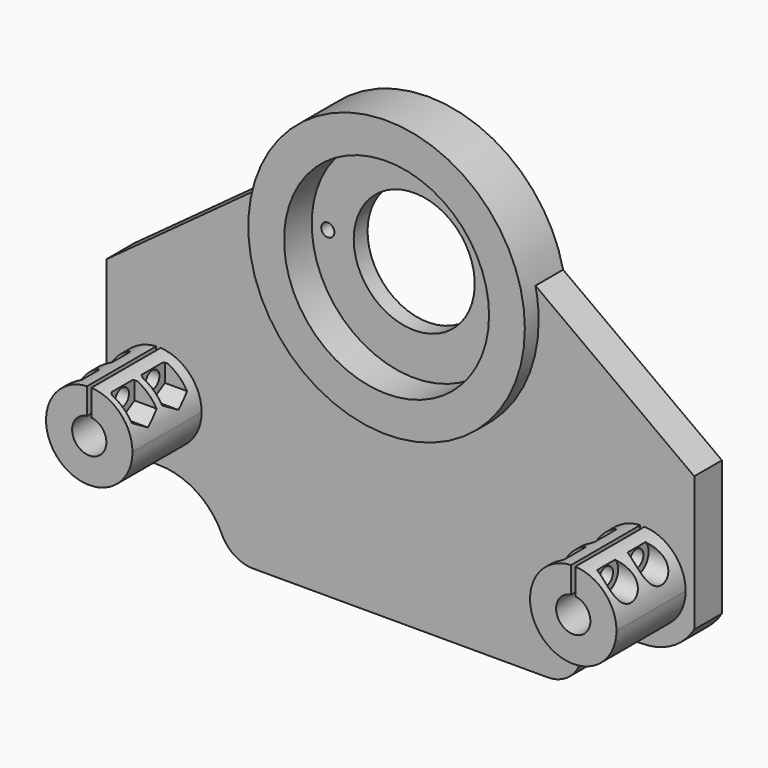
from build123d import *

# Parameters (mm, degrees)
F0_R           = 4.7625
F0_R_2         = 6.2865
F0_R_3         = 37.6555
F1_DEPTH       = 12.7
F2_R           = 63.5
F3_DEPTH       = 25.4
F4_R           = 12.7
F5_R           = 15.875
F5_R_2         = 6.2865
F6_DEPTH       = 31.75
F8_DEPTH       = 31.75
F9_R           = 3.175
F10_DEPTH      = 224.536
F12_DEPTH      = 83.185
F12_DEPTH_BACK = 83.185
F13_R          = 5.55625
F14_DEPTH      = 13.335
F15_R          = 5.55625
F16_DEPTH      = 13.335
F17_W          = 51.1538733715
F17_H          = 19.05
F17_R          = 3.175
F18_DEPTH      = 4.7498
F19_R          = 12.7
F20_R          = 50.8
F20_R_2        = 37.6555
F21_DEPTH      = 12.7
F22_R          = 37.6555
F22_R_2        = 22.225
F23_DEPTH      = 6.35
F24_R          = 2.413
F25_DEPTH      = 25.4
F26_R          = 50.8
F26_R_2        = 37.6555
F27_DEPTH      = 6.35
F29_DEPTH      = 25.4
F29_DEPTH_BACK = 25.4
F31_DEPTH      = 12.7
F32_W          = 127
F32_H          = 63.5
F33_DEPTH      = 12.7
F34_T1_DEPTH   = 12.7
F35_R          = 12.7


# Not quite as in the source:
# - a fillet or chamfer that OpenCascade refuses, or shapes differently, is made with other operations: its cross-section is extruded or revolved along the edge and cut away or added


with BuildPart() as f1:
    # F0 (on Front) → F1 (new body)
    with BuildSketch(Plane.XZ):
        with BuildLine():
            Line((-107.95, 38.1), (-107.95, -69.85))
            Line((-107.95, -69.85), (107.95, -69.85))
            Line((107.95, -69.85), (107.95, 38.1))
            Line((107.95, 38.1), (22.4919418666, 100.6026023463))
            ThreePointArc((22.4919418666, 100.6026023463), (0, 107.95), (-22.4919418666, 100.6026023463))
            Line((-22.4919418666, 100.6026023463), (-107.95, 38.1))
        make_face()
        with Locations((-88.9, -44.45)):
            Circle(F0_R, mode=Mode.SUBTRACT)
        with Locations((-88.9, 0)):
            Circle(F0_R_2, mode=Mode.SUBTRACT)
        with Locations((88.9, -44.45)):
            Circle(F0_R, mode=Mode.SUBTRACT)
        with Locations((88.9, 0)):
            Circle(F0_R_2, mode=Mode.SUBTRACT)
        with Locations((0, 69.85)):
            Circle(F0_R_3, mode=Mode.SUBTRACT)
    extrude(amount=F1_DEPTH)

    # F2 (on face) → F3 (cut)
    with BuildSketch(Plane.XZ.offset(12.7)):
        with Locations((0, -107.95)):
            Circle(F2_R)
    extrude(amount=-F3_DEPTH, mode=Mode.SUBTRACT)

    # F4
    f4_edges = [f1.edges().sort_by_distance(p)[0] for p in [
        (-50.8, -6.35, -69.85),
        (50.8, -6.35, -69.85),
    ]]
    fillet(f4_edges, radius=F4_R)

    # F5 (on face) → F6 (join)
    with BuildSketch(Plane.XZ.offset(12.7)):
        with Locations((-88.9, 0)):
            Circle(F5_R)
        with Locations((-88.9, 0)):
            Circle(F5_R_2, mode=Mode.SUBTRACT)
        with Locations((88.9, 0)):
            Circle(F5_R)
        with Locations((88.9, 0)):
            Circle(F5_R_2, mode=Mode.SUBTRACT)
    extrude(amount=F6_DEPTH)

    # F7 (on face) → F8 (cut, through all)
    with BuildSketch(Plane.XZ.offset(44.45)):
        Polygon((-89.69375, 19.6568928659), (-89.69375, 1.7181718722), (-88.9, 1.7181718722), (-88.10625, 1.7181718722), (-88.10625, 19.6568928659), align=None)
        Polygon((89.69375, 20.8262372762), (88.10625, 20.8262372762), (88.10625, 3.0810327735), (88.9, 3.0810327735), (89.69375, 3.0810327735), align=None)
    extrude(amount=-F8_DEPTH, mode=Mode.SUBTRACT)

    # F9 (on face) → F10 (cut)
    with BuildSketch(Plane(origin=(-107.95, 0, 0), x_dir=(0, -1, 0), z_dir=(-1, 0, 0))):
        with Locations((36.5252, 11.1053438321)):
            Circle(F9_R)
        with Locations((22.5552, 11.1053438321)):
            Circle(F9_R)
    extrude(amount=-F10_DEPTH, mode=Mode.SUBTRACT)

    # F11 (on Right) → F12 (cut, two sides)
    with BuildSketch(Plane.YZ) as f12_sk:
        Polygon((-30.8059682334, 14.4073438321), (-36.5252, 17.7093438321), (-42.2444317666, 14.4073438321), (-42.2444317666, 7.8033438321), (-36.5252, 4.5013438321), (-30.8059682334, 7.8033438321), align=None)
        Polygon((-22.5552, 17.7093438321), (-28.2744317666, 14.4073438321), (-28.2744317666, 7.8033438321), (-22.5552, 4.5013438321), (-16.8359682334, 7.8033438321), (-16.8359682334, 14.4073438321), align=None)
    extrude(amount=-F12_DEPTH, mode=Mode.SUBTRACT)
    extrude(f12_sk.sketch, amount=F12_DEPTH_BACK, mode=Mode.SUBTRACT)

    # F13 (on face) → F14 (cut)
    with BuildSketch(Plane(origin=(-107.95, 0, 0), x_dir=(0, -1, 0), z_dir=(-1, 0, 0))):
        with Locations((22.5552, 11.1053438321)):
            Circle(F13_R)
        with Locations((36.5252, 11.1053438321)):
            Circle(F13_R)
    extrude(amount=-F14_DEPTH, mode=Mode.SUBTRACT)

    # F15 (on face) → F16 (cut)
    with BuildSketch(Plane.YZ.offset(107.95)):
        with Locations((-36.5252, 11.1053438321)):
            Circle(F15_R)
        with Locations((-22.5552, 11.1053438321)):
            Circle(F15_R)
    extrude(amount=-F16_DEPTH, mode=Mode.SUBTRACT)

    # F17 (on face) → F18 (join)
    with BuildSketch(Plane(origin=(0, 0, -69.85), x_dir=(1, 0, 0), z_dir=(0, 0, -1))):
        with Locations((82.3730633142, 22.225)):
            Rectangle(F17_W, F17_H)
        with Locations((82.3730633142, 22.225)):
            Circle(F17_R, mode=Mode.SUBTRACT)
        with Locations((-82.3730633142, 22.225)):
            Rectangle(F17_W, F17_H)
        with Locations((-82.3730633142, 22.225)):
            Circle(F17_R, mode=Mode.SUBTRACT)
    extrude(amount=-F18_DEPTH)

    # F19
    f19_edges = [f1.edges().sort_by_distance(p)[0] for p in [
        (56.796127, -31.75, -67.4751),
        (107.95, -31.75, -67.4751),
        (-56.796127, -31.75, -67.4751),
        (-107.95, -31.75, -67.4751),
    ]]
    fillet(f19_edges, radius=F19_R)

    # F20 (on face) → F21 (join)
    with BuildSketch(Plane.XZ.offset(12.7)):
        with Locations((0, 69.85)):
            Circle(F20_R)
        with Locations((0, 69.85)):
            Circle(F20_R_2, mode=Mode.SUBTRACT)
    extrude(amount=-F21_DEPTH)

    # F22 (on face) → F23 (join)
    with BuildSketch(Plane(origin=(0, 0, 0), x_dir=(-1, 0, 0), z_dir=(0, 1, 0))):
        with Locations((0, 69.85)):
            Circle(F22_R)
        with Locations((0, 69.85)):
            Circle(F22_R_2, mode=Mode.SUBTRACT)
    extrude(amount=-F23_DEPTH)

    # F24 (on face) → F25 (cut)
    with BuildSketch(Plane(origin=(0, 0, 0), x_dir=(-1, 0, 0), z_dir=(0, 1, 0))):
        with Locations((-31.75, 69.7438716888)):
            Circle(F24_R)
        with Locations((31.75, 69.7438716888)):
            Circle(F24_R)
    extrude(amount=-F25_DEPTH, mode=Mode.SUBTRACT)

    # F26 (on face) → F27 (join)
    with BuildSketch(Plane.XZ.offset(12.7)):
        with Locations((0, 69.85)):
            Circle(F26_R)
        with Locations((0, 69.85)):
            Circle(F26_R_2, mode=Mode.SUBTRACT)
    extrude(amount=F27_DEPTH)

    # F28 (on face) → F29 (cut, two sides)
    with BuildSketch(Plane.XZ.offset(12.7)) as f29_sk:
        with BuildLine():
            Line((-111.0971693669, -1.1118889771), (-111.0971693669, 1.1118889771))
            ThreePointArc((-111.0971693669, 1.1118889771), (-111.125, 0), (-111.0971693669, -1.1118889771))
        make_face()
        with BuildLine():
            Line((111.0887860106, 1.268227257), (111.0887860106, -1.268227257))
            ThreePointArc((111.0887860106, -1.268227257), (111.125, 0), (111.0887860106, 1.268227257))
        make_face()
        with BuildLine():
            ThreePointArc((-67.4797934832, -5.9266666667), (-91.3385321133, -22.0908167828), (-111.0971693669, -1.1118889771))
            Line((-111.0971693669, -1.1118889771), (-111.0971693669, -81.4233198762))
            Line((-111.0971693669, -81.4233198762), (111.0887860106, -81.4233198762))
            Line((111.0887860106, -81.4233198762), (111.0887860106, -1.268227257))
            ThreePointArc((111.0887860106, -1.268227257), (91.2607081656, -22.0992688105), (67.4797934832, -5.9266666667))
            ThreePointArc((67.4797934832, -5.9266666667), (58.3800212628, 7.5138896142), (42.999557464, 12.7))
            Line((42.999557464, 12.7), (-42.999557464, 12.7))
            ThreePointArc((-42.999557464, 12.7), (-58.3800212628, 7.5138896142), (-67.4797934832, -5.9266666667))
        make_face()
    extrude(amount=-F29_DEPTH, mode=Mode.SUBTRACT)
    extrude(f29_sk.sketch, amount=F29_DEPTH_BACK, mode=Mode.SUBTRACT)

    # F30 (on face) → F31 (join)
    with BuildSketch(Plane.XZ.offset(12.7)):
        Polygon((60.325, 16.4488966558), (-60.325, 16.4488966558), (-72.7481624406, -10.2908842741), (-88.9, -22.225), (88.9, -22.225), (72.7481624406, -10.2908842741), align=None)
    extrude(amount=-F31_DEPTH)

    # F32 (on face) → F33 (join)
    with BuildSketch(Plane.XZ.offset(12.7)):
        with Locations((0, -12.7)):
            Rectangle(F32_W, F32_H)
    extrude(amount=-F33_DEPTH)

    # F34: fillet of radius 25.4 on 2 edges, made by hand

    # F34_s2 → F34_t1 (join)
    with BuildSketch(Plane.XZ):
        with BuildLine():
            ThreePointArc((-63.5, -44.45), (-71.9002604126, -28.575), (-88.7007812379, -22.225))
            Line((-88.7007812379, -22.225), (-63.5, -22.225))
            Line((-63.5, -22.225), (-63.5, -44.45))
        make_face()
        with BuildLine():
            ThreePointArc((88.7007812379, -22.225), (71.9002604126, -28.575), (63.5, -44.45))
            Line((63.5, -44.45), (63.5, -22.225))
            Line((63.5, -22.225), (88.7007812379, -22.225))
        make_face()
    extrude(amount=F34_T1_DEPTH)

    # F35
    f35_edges = [f1.edges().sort_by_distance(p)[0] for p in [
        (-63.5, -6.35, -44.45),
        (63.5, -6.35, -44.45),
    ]]
    fillet(f35_edges, radius=F35_R)


solid = f1.part
